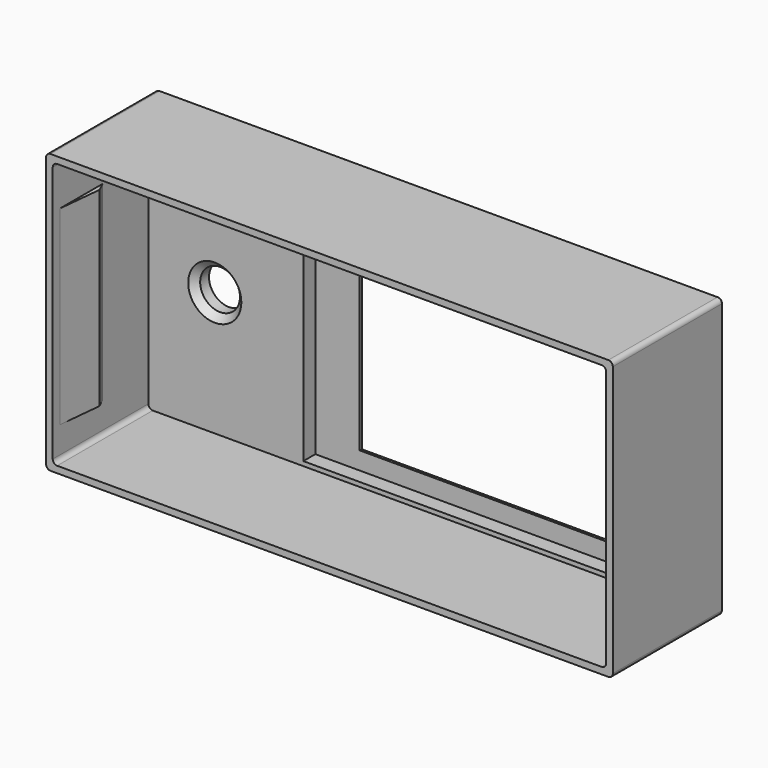
from build123d import *

# Parameters (mm, degrees)
F0_W         = 128
F0_H         = 63
F0_W_2       = 125
F0_H_2       = 60
F1_DEPTH     = 31
F0_R         = 4.5
F0_W_3       = 80
F0_H_3       = 58
F0_W_4       = 65
F0_H_4       = 50
F2_DEPTH     = 4
F3_START     = 0.6
F3_DEPTH     = 3.4
F4_R         = 0.3
F6_START     = 10
F6_DEPTH     = 43
F7_W         = 6
F7_H         = 60
F8_DEPTH     = 1
F9_T1_DEPTH  = 29.5
F9_T3_DEPTH  = 33.5
F9_T6_ANGLE  = 90
F9_T8_ANGLE  = 90
F9_T10_ANGLE = 90
F9_T12_ANGLE = 90
F10_SIZE     = 1.5


# Not quite as in the source:
# - a fillet or chamfer that OpenCascade refuses, or shapes differently, is made with other operations: its cross-section is extruded or revolved along the edge and cut away or added


with BuildPart() as f1:
    # F0 (on Front) → F1 (new body)
    with BuildSketch(Plane.XZ):
        Rectangle(F0_W, F0_H)
        Rectangle(F0_W_2, F0_H_2, mode=Mode.SUBTRACT)
    extrude(amount=F1_DEPTH)

    # F0 (on Front) → F2 (join)
    with BuildSketch(Plane.XZ):
        Rectangle(F0_W_2, F0_H_2)
        with Locations((-47.5, -2)):
            Circle(F0_R, mode=Mode.SUBTRACT)
        with Locations((12.5, 0)):
            Rectangle(F0_W_3, F0_H_3, mode=Mode.SUBTRACT)
        with Locations((12.5, 0)):
            Rectangle(F0_W_3, F0_H_3)
        with Locations((15, 0)):
            Rectangle(F0_W_4, F0_H_4, mode=Mode.SUBTRACT)
    extrude(amount=F2_DEPTH)

    # F0 (on Front) → F3 (cut)
    with BuildSketch(Plane.XZ.offset(F3_START)):
        with Locations((12.5, 0)):
            Rectangle(F0_W_3, F0_H_3)
        with Locations((15, 0)):
            Rectangle(F0_W_4, F0_H_4, mode=Mode.SUBTRACT)
    extrude(amount=F3_DEPTH, mode=Mode.SUBTRACT)

    # F4
    f4_edges = [f1.edges().sort_by_distance(p)[0] for p in [
        (64, 0, 0),
        (0, 0, 31.5),
        (-64, 0, 0),
        (0, 0, -31.5),
    ]]
    fillet(f4_edges, radius=F4_R)

    # F5 (on face) → F6 (join)
    with BuildSketch(Plane(origin=(0, 0, 30), x_dir=(1, 0, 0), z_dir=(0, 0, -1)).offset(F6_START)):
        Polygon((-61.5, 19.0501256289), (-62.5, 29), (-62.5, 16.9056187084), align=None)
        Polygon((62.5, 16.9056187084), (62.5, 29), (61.5, 19.0501256289), align=None)
    extrude(amount=F6_DEPTH)

    # F7 (on face) → F8 (join)
    with BuildSketch(Plane.XZ):
        with Locations((-30.5, 0)):
            Rectangle(F7_W, F7_H)
        with Locations((55.5, 0)):
            Rectangle(F7_W, F7_H)
    extrude(amount=F8_DEPTH)

    # F9: fillet of radius 1 on 8 edges, made by hand

    # F9_s2 → F9_t1 (join)
    with BuildSketch(Plane.XZ.offset(1.5)):
        with BuildLine():
            ThreePointArc((62.5, 29), (62.2071067812, 29.7071067812), (61.5, 30))
            Line((61.5, 30), (62.5, 30))
            Line((62.5, 30), (62.5, 29))
        make_face()
        with BuildLine():
            ThreePointArc((-62.5, 29), (-62.2071067812, 29.7071067812), (-61.5, 30))
            Line((-61.5, 30), (-62.5, 30))
            Line((-62.5, 30), (-62.5, 29))
        make_face()
        with BuildLine():
            ThreePointArc((-61.5, -30), (-62.2071067812, -29.7071067812), (-62.5, -29))
            Line((-62.5, -29), (-62.5, -30))
            Line((-62.5, -30), (-61.5, -30))
        make_face()
        with BuildLine():
            ThreePointArc((61.5, -30), (62.2071067812, -29.7071067812), (62.5, -29))
            Line((62.5, -29), (62.5, -30))
            Line((62.5, -30), (61.5, -30))
        make_face()
    extrude(amount=F9_T1_DEPTH)

    # F9_s4 → F9_t3 (cut)
    with BuildSketch(Plane.XZ):
        with BuildLine():
            ThreePointArc((63, 31.5), (63.7071067812, 31.2071067812), (64, 30.5))
            Line((64, 30.5), (64, 31.5))
            Line((64, 31.5), (63, 31.5))
        make_face()
        with BuildLine():
            ThreePointArc((64, -30.5), (63.7071067812, -31.2071067812), (63, -31.5))
            Line((63, -31.5), (64, -31.5))
            Line((64, -31.5), (64, -30.5))
        make_face()
        with BuildLine():
            ThreePointArc((-63, 31.5), (-63.7071067812, 31.2071067812), (-64, 30.5))
            Line((-64, 30.5), (-64, 31.5))
            Line((-64, 31.5), (-63, 31.5))
        make_face()
        with BuildLine():
            ThreePointArc((-64, -30.5), (-63.7071067812, -31.2071067812), (-63, -31.5))
            Line((-63, -31.5), (-64, -31.5))
            Line((-64, -31.5), (-64, -30.5))
        make_face()
    extrude(amount=F9_T3_DEPTH, mode=Mode.SUBTRACT)

    # F9_s5 → F9_t6 (revolve, cut)
    with BuildSketch(Plane.YZ.offset(-63)):
        with BuildLine():
            ThreePointArc((0, -31.2), (-0.0878679656, -31.4121320344), (-0.3, -31.5))
            Line((-0.3, -31.5), (0, -31.5))
            Line((0, -31.5), (0, -31.2))
        make_face()
    revolve(axis=Axis((-63, 0, -30.5), (0, 1, 0)), revolution_arc=F9_T6_ANGLE, mode=Mode.SUBTRACT)

    # F9_s7 → F9_t8 (revolve, cut)
    with BuildSketch(Plane.XY.offset(30.5)):
        with BuildLine():
            ThreePointArc((-63.7, 0), (-63.9121320344, -0.0878679656), (-64, -0.3))
            Line((-64, -0.3), (-64, 0))
            Line((-64, 0), (-63.7, 0))
        make_face()
    revolve(axis=Axis((-63, 0, 30.5), (0, 1, 0)), revolution_arc=F9_T8_ANGLE, mode=Mode.SUBTRACT)

    # F9_s9 → F9_t10 (revolve, cut)
    with BuildSketch(Plane.XY.offset(-30.5)):
        with BuildLine():
            ThreePointArc((63.7, 0), (63.9121320344, -0.0878679656), (64, -0.3))
            Line((64, -0.3), (64, 0))
            Line((64, 0), (63.7, 0))
        make_face()
    revolve(axis=Axis((63, 0, -30.5), (0, 1, 0)), revolution_arc=F9_T10_ANGLE, mode=Mode.SUBTRACT)

    # F9_s11 → F9_t12 (revolve, cut)
    with BuildSketch(Plane.YZ.offset(63)):
        with BuildLine():
            ThreePointArc((0, 31.2), (-0.0878679656, 31.4121320344), (-0.3, 31.5))
            Line((-0.3, 31.5), (0, 31.5))
            Line((0, 31.5), (0, 31.2))
        make_face()
    revolve(axis=Axis((63, 0, 30.5), (0, 1, 0)), revolution_arc=F9_T12_ANGLE, mode=Mode.SUBTRACT)

    # F10
    f10_edges = [f1.edges().sort_by_distance(p)[0] for p in [
        (-52, -4, -2),
    ]]
    chamfer(f10_edges, length=F10_SIZE)


solid = f1.part
